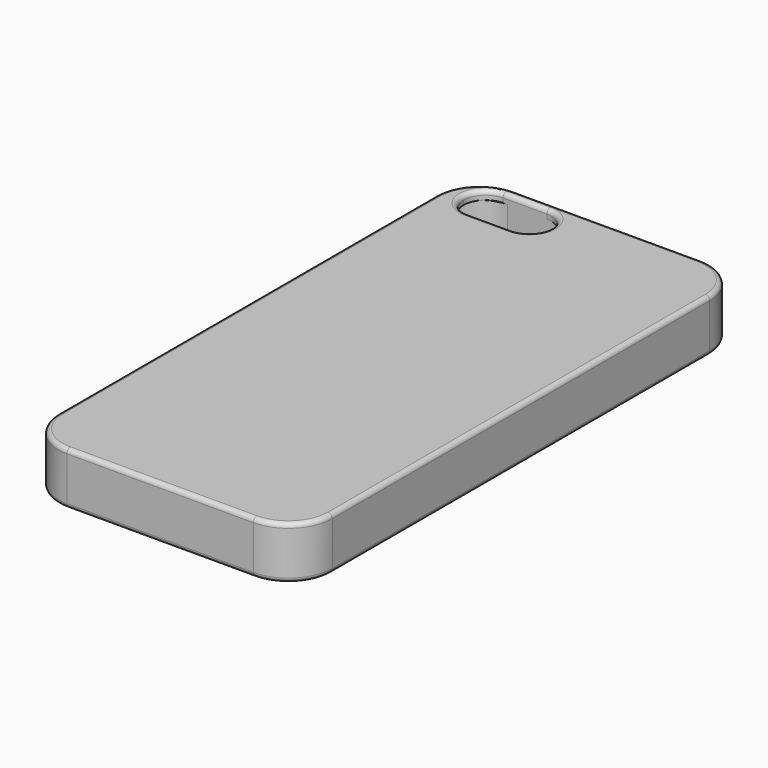
from build123d import *

# Parameters (mm, degrees)
F1_DEPTH     = 2
F3_DEPTH     = 10
F5_DEPTH     = 2
F6_R         = 1
F7_R         = 0.99999
F8_R         = 1
F9_T1_DEPTH  = 42.6
F9_T3_DEPTH  = 107.8
F9_T5_DEPTH  = 10
F9_T8_ANGLE  = 90
F9_T10_ANGLE = 90
F9_T12_ANGLE = 90
F9_T14_ANGLE = 90
F9_T16_ANGLE = 180
F9_T18_ANGLE = 180


# Not quite as in the source:
# - a fillet or chamfer that OpenCascade refuses, or shapes differently, is made with other operations: its cross-section is extruded or revolved along the edge and cut away or added
# - a fillet or chamfer is up to 0.001 mm smaller than in the source, because OpenCascade refuses the exact size


with BuildPart() as f1:
    # F0 (on Top) → F1 (new body)
    with BuildSketch(Plane.XY):
        with BuildLine():
            ThreePointArc((0, 10), (2.9289321881, 2.9289321881), (10, 0))
            Line((10, 0), (52.6, 0))
            ThreePointArc((52.6, 0), (59.6710678119, 2.9289321881), (62.6, 10))
            Line((62.6, 10), (62.6, 117.8))
            ThreePointArc((62.6, 117.8), (59.6710678119, 124.8710678119), (52.6, 127.8))
            Line((52.6, 127.8), (10, 127.8))
            ThreePointArc((10, 127.8), (2.9289321881, 124.8710678119), (0, 117.8))
            Line((0, 117.8), (0, 10))
        make_face()
        with BuildLine():
            ThreePointArc((4, 120.8), (5.4644660941, 124.3355339059), (9, 125.8))
            Line((9, 125.8), (19, 125.8))
            ThreePointArc((19, 125.8), (22.5355339059, 124.3355339059), (24, 120.8))
            ThreePointArc((24, 120.8), (22.5355339059, 117.2644660941), (19, 115.8))
            Line((19, 115.8), (9, 115.8))
            ThreePointArc((9, 115.8), (5.4644660941, 117.2644660941), (4, 120.8))
        make_face(mode=Mode.SUBTRACT)
    extrude(amount=F1_DEPTH)

    # F2 (on Top) → F3 (join)
    with BuildSketch(Plane.XY):
        with BuildLine():
            ThreePointArc((0, 10), (2.9289321881, 2.9289321881), (10, 0))
            Line((10, 0), (52.6, 0))
            ThreePointArc((52.6, 0), (59.6710678119, 2.9289321881), (62.6, 10))
            Line((62.6, 10), (62.6, 117.8))
            ThreePointArc((62.6, 117.8), (59.6710678119, 124.8710678119), (52.6, 127.8))
            Line((52.6, 127.8), (10, 127.8))
            ThreePointArc((10, 127.8), (2.9289321881, 124.8710678119), (0, 117.8))
            Line((0, 117.8), (0, 10))
        make_face()
        with BuildLine():
            ThreePointArc((10, 2), (4.3431457505, 4.3431457505), (2, 10))
            Line((2, 10), (2, 117.8))
            ThreePointArc((2, 117.8), (4.3431457505, 123.4568542495), (10, 125.8))
            Line((10, 125.8), (52.6, 125.8))
            ThreePointArc((52.6, 125.8), (58.2568542495, 123.4568542495), (60.6, 117.8))
            Line((60.6, 117.8), (60.6, 10))
            ThreePointArc((60.6, 10), (58.2568542495, 4.3431457505), (52.6, 2))
            Line((52.6, 2), (10, 2))
        make_face(mode=Mode.SUBTRACT)
    extrude(amount=-F3_DEPTH)

    # F4 (on face) → F5 (join)
    with BuildSketch(Plane(origin=(0, 0, -10), x_dir=(1, 0, 0), z_dir=(0, 0, -1))):
        with BuildLine():
            ThreePointArc((0, -117.8), (2.9289321881, -124.8710678119), (10, -127.8))
            Line((10, -127.8), (52.6, -127.8))
            ThreePointArc((52.6, -127.8), (59.6710678119, -124.8710678119), (62.6, -117.8))
            Line((62.6, -117.8), (62.6, -10))
            ThreePointArc((62.6, -10), (59.6710678119, -2.9289321881), (52.6, 0))
            Line((52.6, 0), (10, 0))
            ThreePointArc((10, 0), (2.9289321881, -2.9289321881), (0, -10))
            Line((0, -10), (0, -117.8))
        make_face()
        with BuildLine():
            ThreePointArc((10, -124.8), (5.0502525317, -122.7497474683), (3, -117.8))
            Line((3, -117.8), (3, -10))
            ThreePointArc((3, -10), (5.0502525317, -5.0502525317), (10, -3))
            Line((10, -3), (52.6, -3))
            ThreePointArc((52.6, -3), (57.5497474683, -5.0502525317), (59.6, -10))
            Line((59.6, -10), (59.6, -117.8))
            ThreePointArc((59.6, -117.8), (57.5497474683, -122.7497474683), (52.6, -124.8))
            Line((52.6, -124.8), (10, -124.8))
        make_face(mode=Mode.SUBTRACT)
    extrude(amount=-F5_DEPTH)

    # F6
    f6_edges = [f1.edges().sort_by_distance(p)[0] for p in [
        (31.3, 124.8, -10),
    ]]
    fillet(f6_edges, radius=F6_R)

    # F7 (radius 1 in the source; OpenCascade refuses exactly that, so slightly less here)
    f7_edges = [f1.edges().sort_by_distance(p)[0] for p in [
        (31.3, 124.8, -8),
        (57.549747, 122.749747, -8),
        (59.6, 63.9, -8),
        (57.549747, 5.050253, -8),
        (31.3, 3, -8),
        (5.050253, 5.050253, -8),
        (3, 63.9, -8),
        (5.050253, 122.749747, -8),
    ]]
    fillet(f7_edges, radius=F7_R)

    # F8
    f8_edges = [f1.edges().sort_by_distance(p)[0] for p in [
        (62.6, 63.9, -10),
        (59.671068, 124.871068, -10),
        (31.3, 127.8, -10),
        (2.928932, 124.871068, -10),
        (0, 63.9, -10),
        (2.928932, 2.928932, -10),
        (31.3, 0, -10),
        (59.671068, 2.928932, -10),
    ]]
    fillet(f8_edges, radius=F8_R)

    # F9: fillet of radius 1 on 12 edges, made by hand

    # F9_s2 → F9_t1 (cut)
    with BuildSketch(Plane.YZ.offset(10)):
        with BuildLine():
            ThreePointArc((0, 1), (0.2928932188, 1.7071067812), (1, 2))
            Line((1, 2), (0, 2))
            Line((0, 2), (0, 1))
        make_face()
        with BuildLine():
            ThreePointArc((127.8, 1), (127.5071067812, 1.7071067812), (126.8, 2))
            Line((126.8, 2), (127.8, 2))
            Line((127.8, 2), (127.8, 1))
        make_face()
    extrude(amount=F9_T1_DEPTH, mode=Mode.SUBTRACT)

    # F9_s4 → F9_t3 (cut)
    with BuildSketch(Plane.XZ.offset(-117.8)):
        with BuildLine():
            ThreePointArc((0, 1), (0.2928932188, 1.7071067812), (1, 2))
            Line((1, 2), (0, 2))
            Line((0, 2), (0, 1))
        make_face()
        with BuildLine():
            ThreePointArc((62.6, 1), (62.3071067812, 1.7071067812), (61.6, 2))
            Line((61.6, 2), (62.6, 2))
            Line((62.6, 2), (62.6, 1))
        make_face()
    extrude(amount=F9_T3_DEPTH, mode=Mode.SUBTRACT)

    # F9_s6 → F9_t5 (cut)
    with BuildSketch(Plane.YZ.offset(9)):
        with BuildLine():
            ThreePointArc((126.8, 2), (126.0928932188, 1.7071067812), (125.8, 1))
            Line((125.8, 1), (125.8, 2))
            Line((125.8, 2), (126.8, 2))
        make_face()
        with BuildLine():
            ThreePointArc((114.8, 2), (115.5071067812, 1.7071067812), (115.8, 1))
            Line((115.8, 1), (115.8, 2))
            Line((115.8, 2), (114.8, 2))
        make_face()
    extrude(amount=F9_T5_DEPTH, mode=Mode.SUBTRACT)

    # F9_s7 → F9_t8 (revolve, cut)
    with BuildSketch(Plane.XZ.offset(-10)):
        with BuildLine():
            ThreePointArc((0, 1), (0.2928932188, 1.7071067812), (1, 2))
            Line((1, 2), (0, 2))
            Line((0, 2), (0, 1))
        make_face()
    revolve(axis=Axis((10, 10, 2), (0, 0, 1)), revolution_arc=F9_T8_ANGLE, mode=Mode.SUBTRACT)

    # F9_s9 → F9_t10 (revolve, cut)
    with BuildSketch(Plane.YZ.offset(52.6)):
        with BuildLine():
            ThreePointArc((0, 1), (0.2928932188, 1.7071067812), (1, 2))
            Line((1, 2), (0, 2))
            Line((0, 2), (0, 1))
        make_face()
    revolve(axis=Axis((52.6, 10, 2), (0, 0, 1)), revolution_arc=F9_T10_ANGLE, mode=Mode.SUBTRACT)

    # F9_s11 → F9_t12 (revolve, cut)
    with BuildSketch(Plane.XZ.offset(-117.8)):
        with BuildLine():
            ThreePointArc((62.6, 1), (62.3071067812, 1.7071067812), (61.6, 2))
            Line((61.6, 2), (62.6, 2))
            Line((62.6, 2), (62.6, 1))
        make_face()
    revolve(axis=Axis((52.6, 117.8, 2), (0, 0, 1)), revolution_arc=F9_T12_ANGLE, mode=Mode.SUBTRACT)

    # F9_s13 → F9_t14 (revolve, cut)
    with BuildSketch(Plane.YZ.offset(10)):
        with BuildLine():
            ThreePointArc((127.8, 1), (127.5071067812, 1.7071067812), (126.8, 2))
            Line((126.8, 2), (127.8, 2))
            Line((127.8, 2), (127.8, 1))
        make_face()
    revolve(axis=Axis((10, 117.8, 2), (0, 0, 1)), revolution_arc=F9_T14_ANGLE, mode=Mode.SUBTRACT)

    # F9_s15 → F9_t16 (revolve, cut)
    with BuildSketch(Plane.YZ.offset(9)):
        with BuildLine():
            ThreePointArc((126.8, 2), (126.0928932188, 1.7071067812), (125.8, 1))
            Line((125.8, 1), (125.8, 2))
            Line((125.8, 2), (126.8, 2))
        make_face()
    revolve(axis=Axis((9, 120.8, 2), (0, 0, 1)), revolution_arc=F9_T16_ANGLE, mode=Mode.SUBTRACT)

    # F9_s17 → F9_t18 (revolve, cut)
    with BuildSketch(Plane.YZ.offset(19)):
        with BuildLine():
            ThreePointArc((114.8, 2), (115.5071067812, 1.7071067812), (115.8, 1))
            Line((115.8, 1), (115.8, 2))
            Line((115.8, 2), (114.8, 2))
        make_face()
    revolve(axis=Axis((19, 120.8, 2), (0, 0, 1)), revolution_arc=F9_T18_ANGLE, mode=Mode.SUBTRACT)


solid = f1.part
